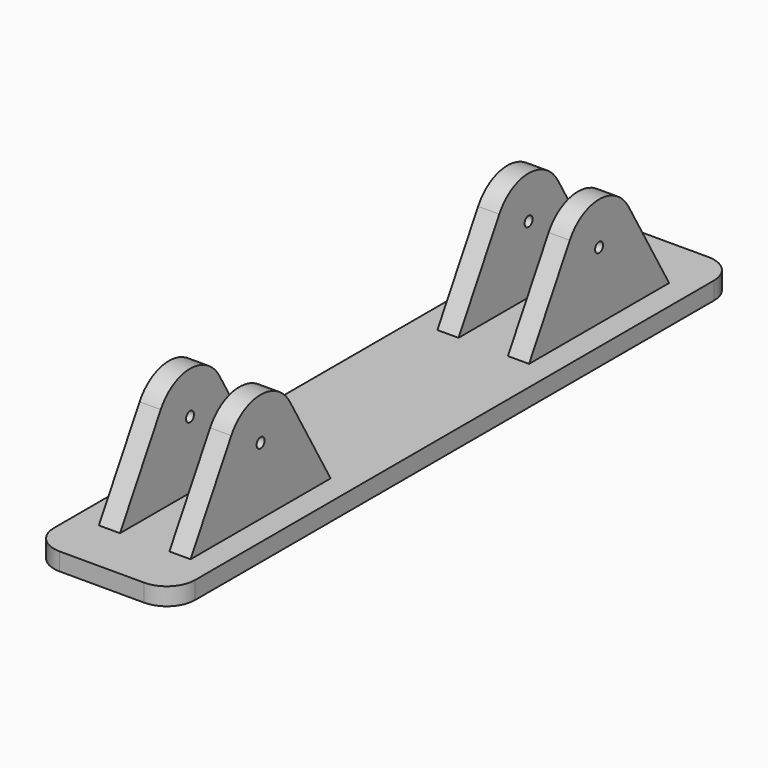
from build123d import *

# Parameters (mm, degrees)
F0_W     = 25.4
F0_H     = 127
F1_DEPTH = 3.175
F3_DEPTH = 8.255
F4_DEPTH = 4.445
F5_R     = 0.9
F6_DEPTH = 20.956
F7_R     = 5.08


# Not quite as in the source:
# - a pattern or mirror of a feature is missing from the dataset's text; its kind, count and spacing are read off the source's solid


with BuildPart() as f1:
    # F0 (on Top) → F1 (new body)
    with BuildSketch(Plane.XY):
        Rectangle(F0_W, F0_H)
    extrude(amount=F1_DEPTH)

    # F2 (on Right) → F3 (join, symmetric)
    with BuildSketch(Plane.YZ):
        with BuildLine():
            Line((-44.6991135768, 19.05), (-53.8645491002, 3.175))
            Line((-53.8645491002, 3.175), (-22.3354508998, 3.175))
            Line((-22.3354508998, 3.175), (-31.5008864232, 19.05))
            ThreePointArc((-31.5008864232, 19.05), (-38.1, 22.86), (-44.6991135768, 19.05))
        make_face()
    f3 = extrude(amount=F3_DEPTH, both=True)

    # F3_copies: F3 across plane
    add(f3.mirror(Plane.ZX))

    # F2 (on Right) → F4 (cut, symmetric)
    with BuildSketch(Plane.YZ):
        with BuildLine():
            Line((-44.6991135768, 19.05), (-53.8645491002, 3.175))
            Line((-53.8645491002, 3.175), (-22.3354508998, 3.175))
            Line((-22.3354508998, 3.175), (-31.5008864232, 19.05))
            ThreePointArc((-31.5008864232, 19.05), (-38.1, 22.86), (-44.6991135768, 19.05))
        make_face()
    f4 = extrude(amount=F4_DEPTH, both=True, mode=Mode.SUBTRACT)

    # F4_copies: F4 across plane
    add(f4.mirror(Plane.ZX), mode=Mode.SUBTRACT)

    # F5 (on face) → F6 (cut, through all)
    with BuildSketch(Plane.YZ.offset(8.255)):
        with Locations((-38.1, 15.24)):
            Circle(F5_R)
    f6 = extrude(amount=-F6_DEPTH, mode=Mode.SUBTRACT)

    # F6_copies: F6 across plane
    add(f6.mirror(Plane.ZX), mode=Mode.SUBTRACT)

    # F7
    f7_edges = [f1.edges().sort_by_distance(p)[0] for p in [
        (12.7, -63.5, 1.5875),
        (-12.7, -63.5, 1.5875),
        (12.7, 63.5, 1.5875),
        (-12.7, 63.5, 1.5875),
    ]]
    fillet(f7_edges, radius=F7_R)


solid = f1.part
